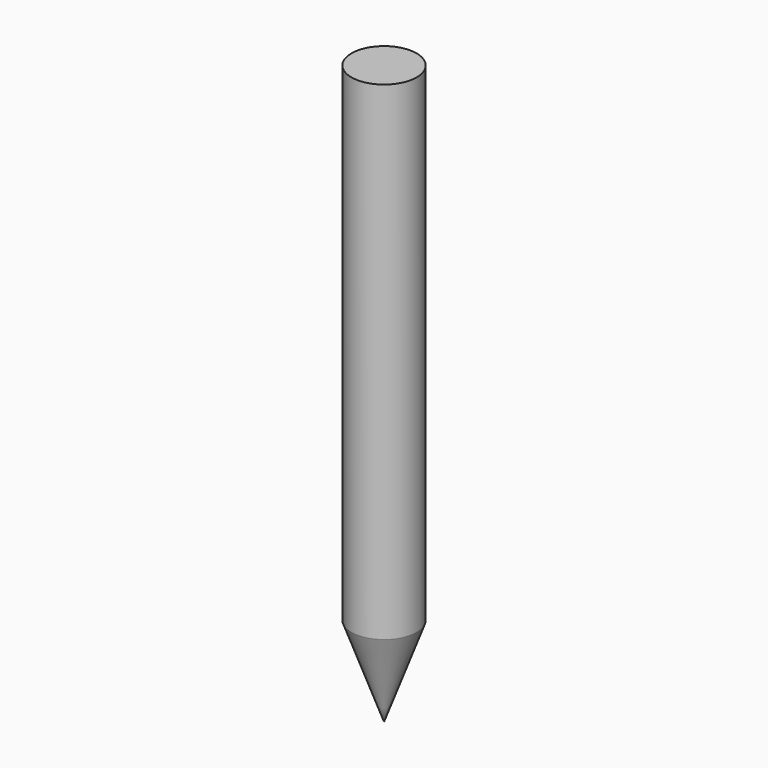
from build123d import *

# Parameters (mm, degrees)
F0_R     = 2
F1_DEPTH = 30


# Not quite as in the source:
# - an extrude whose draft closes it to a point is written as a loft to that point


with BuildPart() as f1:
    # F0 (on Top) → F1 (new body)
    with BuildSketch(Plane.XY):
        Circle(F0_R)
    extrude(amount=F1_DEPTH)

    # F0 (on Top) → F2 section 0
    with BuildSketch(Plane.XY, mode=Mode.PRIVATE) as f2_s0:
        Circle(F0_R)
    loft([f2_s0.sketch, Vertex(0, 0, -5.4949548389)], ruled=True)


solid = f1.part
